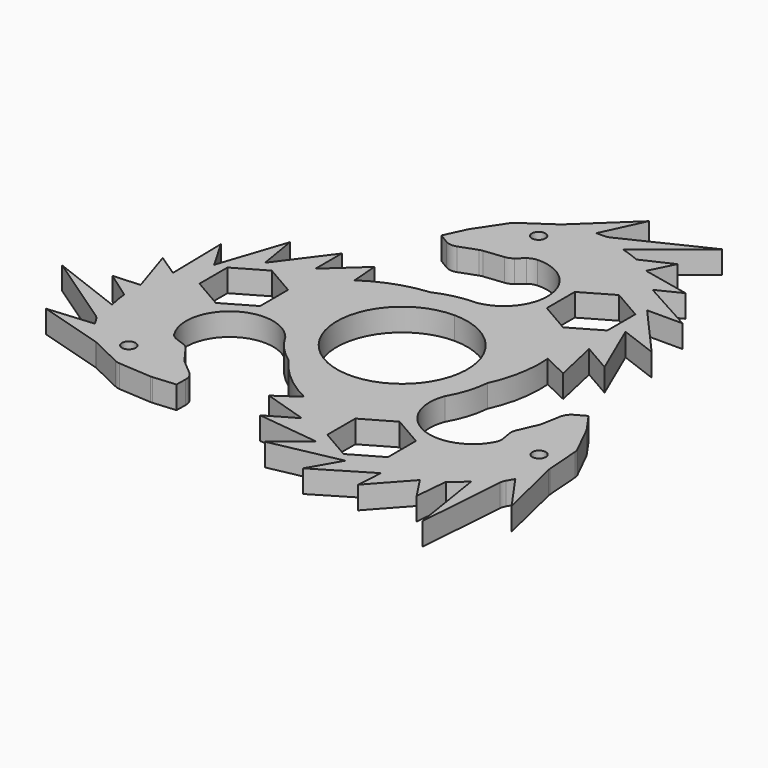
from build123d import *

# Parameters (mm, degrees)
F0_R     = 1.5
F1_DEPTH = 5
F3_COUNT = 3


# Not quite as in the source:
# - a feature names something its author has since deleted; it is built from what else it names


with BuildPart() as f1:
    # F0 (on Top) → F1 (new body)
    with BuildSketch(Plane.XY):
        with BuildLine():
            ThreePointArc((-1.7478732612, 39.5149783142), (8.1392001596, 30.7821912097), (0, 20.4009960858))
            Line((0, 20.4009960858), (0, 14.4152096754))
            ThreePointArc((0, 14.4152096754), (12.4839377798, 7.2076048377), (12.4839377798, -7.2076048377))
            Line((12.4839377798, -7.2076048377), (17.6677808728, -10.2004980429))
            ThreePointArc((17.6677808728, -10.2004980429), (19.4452285789, -6.171201407), (20.3165472355, -1.8543326892))
            ThreePointArc((20.3165472355, -1.8543326892), (22.4085751719, 4.7991946551), (22.7576271971, 11.7651238603))
            Line((22.7576271971, 11.7651238603), (28.2481051981, 9.1530177742))
            Line((28.2481051981, 9.1530177742), (26.0387565941, 19.0982837094))
            Line((26.0387565941, 19.0982837094), (32.3511809111, 15.4654439539))
            Line((32.3511809111, 15.4654439539), (26.9242947963, 28.0441137764))
            Line((26.9242947963, 28.0441137764), (35.1917743683, 24.9340832233))
            Line((35.1917743683, 24.9340832233), (24.8427105993, 36.6120710969))
            Line((24.8427105993, 36.6120710969), (32.6668024063, 36.6120710969))
            Line((32.6668024063, 36.6120710969), (20.8077298225, 43.1800760308))
            Line((20.8077298225, 43.1800760308), (26.0387565941, 45.7650870085))
            Line((26.0387565941, 45.7650870085), (15.485866915, 48.02231204))
            Line((15.485866915, 48.02231204), (18.1482266635, 53.3400028944))
            Line((18.1482266635, 53.3400028944), (11.520179105, 50.2734731867))
            ThreePointArc((11.520179105, 50.2734731867), (9.4992839441, 51.1021592503), (7.4171009474, 51.7618954182))
            Line((7.4171009474, 51.7618954182), (20.6731967628, 62.493018806))
            Line((20.6731967628, 62.493018806), (2.9851620813, 53.9539658583))
            ThreePointArc((2.9851620813, 53.9539658583), (2.3498823759, 53.7311579429), (1.6809146705, 53.6556206644))
            Line((1.6809146705, 53.6556206644), (0, 53.6556206644))
            Line((0, 53.6556206644), (4.2608887888, 62.8086403012))
            Line((4.2608887888, 62.8086403012), (-6.6135251858, 52.5556231266))
            ThreePointArc((-6.6135251858, 52.5556231266), (-6.7917072446, 52.4004137483), (-6.9815525166, 52.2597099106))
            Line((-6.9815525166, 52.2597099106), (-13.2472028108, 47.9876733272))
            ThreePointArc((-13.2472028108, 47.9876733272), (-13.6895314092, 47.6192351761), (-14.0533422232, 47.1730928761))
            Line((-14.0533422232, 47.1730928761), (-18.0220315222, 41.2200618552))
            ThreePointArc((-18.0220315222, 41.2200618552), (-18.1407171431, 41.0265497088), (-18.2444304369, 40.824617096))
            Line((-18.2444304369, 40.824617096), (-20.3575752676, 36.2964496017))
            Line((-20.3575752676, 36.2964496017), (-18.2173253559, 35.0123005809))
            ThreePointArc((-18.2173253559, 35.0123005809), (-16.9608718875, 34.5985427406), (-15.6486105692, 34.7653992696))
            Line((-15.6486105692, 34.7653992696), (-11.8852458251, 36.1338942554))
            ThreePointArc((-11.8852458251, 36.1338942554), (-11.5431146027, 36.2357083507), (-11.1913122519, 36.2961648589))
            Line((-11.1913122519, 36.2961648589), (-6.7715043443, 36.7872549082))
            ThreePointArc((-6.7715043443, 36.7872549082), (-5.920047927, 37.0118969078), (-5.1704976221, 37.4740834492))
            Line((-5.1704976221, 37.4740834492), (-3.5822876233, 38.8113983631))
            ThreePointArc((-3.5822876233, 38.8113983631), (-2.7243104061, 39.3176161279), (-1.7478732612, 39.5149783142))
        make_face()
        with Locations((-7.1445683185, 46.6340765733)):
            Circle(F0_R, mode=Mode.SUBTRACT)
        Polygon((10.8037195943, 34.1769884273), (17.5, 38.0430877221), (24.1962804057, 34.1769884273), (24.1962804057, 26.4447898377), (17.5, 22.5786905429), (10.8037195943, 26.4447898377), align=None, mode=Mode.SUBTRACT)
    extrude(amount=F1_DEPTH)

    # F3: F1 ×3 about axis
    f3_axis = Axis((0, 0, 21.8280367553), (0, 0, 1))


with BuildPart() as f1_1:
    add(f1.part)
    for i in range(1, F3_COUNT):
        add(f1.part.rotate(f3_axis, i * 360 / F3_COUNT))


solid = f1_1.part
